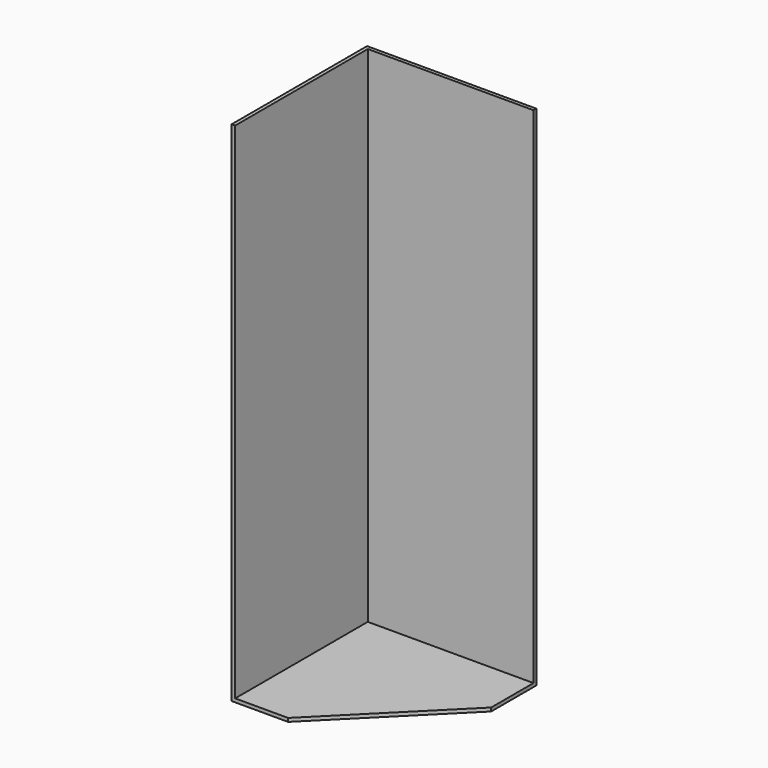
from build123d import *

# Parameters (mm, degrees)
F0_W     = 609.6
F0_H     = 1828.8
F1_DEPTH = 12.7
F4_W     = 596.9
F4_H     = 596.9
F5_DEPTH = 12.7
F6_SIZE  = 406.4


# Not quite as in the source:
# - a feature of the source that left no trace in its solid (it failed there, or was rolled back) is left out
# - a pattern or mirror of a feature is missing from the dataset's text; its kind, count and spacing are read off the source's solid


with BuildPart() as f1:
    # F0 (on Front) → F1 (new body)
    with BuildSketch(Plane.XZ):
        with Locations((304.8, 85.8015570831)):
            Rectangle(F0_W, F0_H)
    extrude(amount=F1_DEPTH)

    # F1_copies: F1 across plane


with BuildPart() as f1_1:
    add(f1.part)
    add(f1.part.mirror(Plane(origin=(0, 0, 0), x_dir=(0.7071067812, -0.7071067812, 0), z_dir=(-0.7071067812, -0.7071067812, 0))))

    # F4 (on face) → F5 (join)
    with BuildSketch(Plane(origin=(0, 0, -828.5984429169), x_dir=(1, 0, 0), z_dir=(0, 0, -1))):
        with Locations((311.15, 311.15)):
            Rectangle(F4_W, F4_H)
    extrude(amount=-F5_DEPTH)

    # F6
    f6_edges = [f1_1.edges().sort_by_distance(p)[0] for p in [
        (609.6, -609.6, -822.248443),
    ]]
    chamfer(f6_edges, length=F6_SIZE)


solid = f1_1.part
